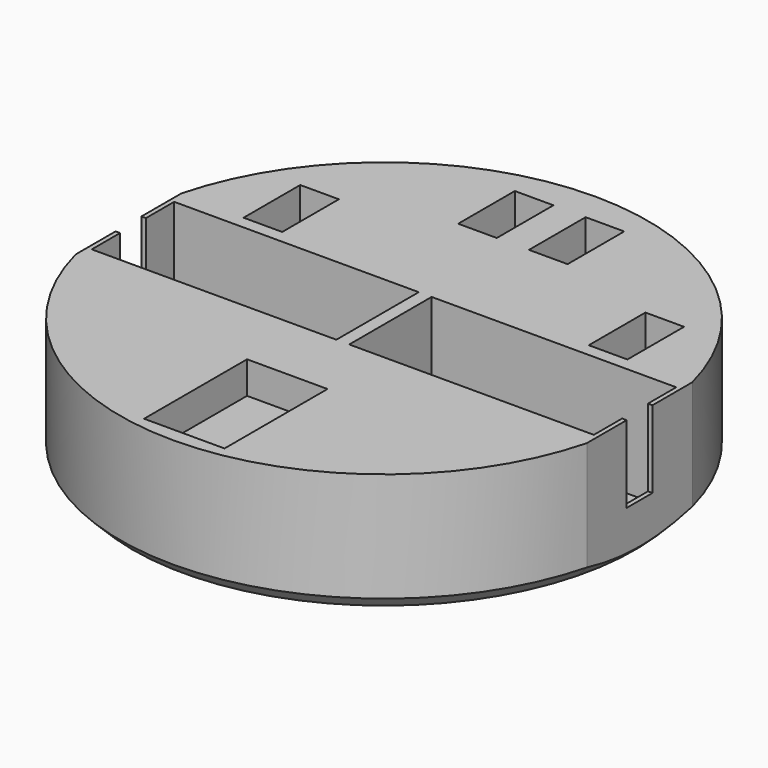
from build123d import *

# Parameters (mm, degrees)
F0_R        = 41
F1_DEPTH    = 19
F3_DEPTH    = 17
F4_W        = 6
F4_H        = 11
F4_W_2      = 11
F4_H_2      = 16
F4_W_3      = 10.7800960541
F4_H_3      = 45.1917052269
F5_DEPTH    = 19.001
F7_START    = -12
F6_W        = 0.7
F6_H        = 5
F7_DEPTH    = 5
F8_W        = 16
F8_H        = 16
F9_DEPTH    = 1.82
F10_C1_SIZE = 2
F10_C2_SIZE = 1.9999
F11_W       = 12.5
F11_H       = 20
F12_DEPTH   = 5
F13_W       = 6
F13_H       = 35
F14_DEPTH   = 28.5


# Not quite as in the source:
# - a fillet or chamfer is up to 0.001 mm smaller than in the source, because OpenCascade refuses the exact size


with BuildPart() as f1:
    # F0 (on Top) → F1 (new body)
    with BuildSketch(Plane.XY):
        Circle(F0_R)
    extrude(amount=F1_DEPTH)

    # F2 (on face) → F3 (cut)
    with BuildSketch(Plane.XY.offset(19)):
        Polygon((39, 2.5), (39, 8), (1, 8), (1, -8), (39, -8), (39, -2.5), align=None)
        Polygon((-39, 8), (-39, 2.5), (-39, -2.5), (-39, -8), (-1, -8), (-1, 8), align=None)
        with BuildLine():
            Line((43, 2.5), (40.9237095093, 2.5))
            ThreePointArc((40.9237095093, 2.5), (40.9809229391, 1.2505818885), (41, 0))
            ThreePointArc((41, 0), (40.9809229391, -1.2505818885), (40.9237095093, -2.5))
            Line((40.9237095093, -2.5), (43, -2.5))
            Line((43, -2.5), (43, 2.5))
        make_face()
        with BuildLine():
            ThreePointArc((-40.9237095093, -2.5), (-41, 0), (-40.9237095093, 2.5))
            Line((-40.9237095093, 2.5), (-43, 2.5))
            Line((-43, 2.5), (-43, -2.5))
            Line((-43, -2.5), (-40.9237095093, -2.5))
        make_face()
        with BuildLine():
            Line((40.9237095093, 2.5), (39, 2.5))
            Line((39, 2.5), (39, -2.5))
            Line((39, -2.5), (40.9237095093, -2.5))
            ThreePointArc((40.9237095093, -2.5), (40.9809229391, -1.2505818885), (41, 0))
            ThreePointArc((41, 0), (40.9809229391, 1.2505818885), (40.9237095093, 2.5))
        make_face()
        with BuildLine():
            Line((-39, 2.5), (-40.9237095093, 2.5))
            ThreePointArc((-40.9237095093, 2.5), (-41, 0), (-40.9237095093, -2.5))
            Line((-40.9237095093, -2.5), (-39, -2.5))
            Line((-39, -2.5), (-39, 2.5))
        make_face()
    extrude(amount=-F3_DEPTH, mode=Mode.SUBTRACT)

    # F4 (on face) → F5 (cut, through all)
    with BuildSketch(Plane.XY.offset(19)):
        with Locations((-26.8149985671, 15.5)):
            Rectangle(F4_W, F4_H)
        with Locations((26.8149985671, 15.5)):
            Rectangle(F4_W, F4_H)
        with Locations((-5.5, 30.5270385295)):
            Rectangle(F4_W, F4_H)
        with Locations((5.5, 30.5270385295)):
            Rectangle(F4_W, F4_H)
        with Locations((-6.5, 0)):
            Rectangle(F4_W_2, F4_H_2)
        with Locations((6.5, 0)):
            Rectangle(F4_W_2, F4_H_2)
        with Locations((-45.090048027, 0)):
            Rectangle(F4_W_3, F4_H_3)
        with Locations((45.090048027, 0)):
            Rectangle(F4_W_3, F4_H_3)
    extrude(amount=-F5_DEPTH, mode=Mode.SUBTRACT)

    # F6 (on face) → F7 (join)
    with BuildSketch(Plane.XY.offset(19).offset(F7_START)):
        with Locations((-39.35, 0)):
            Rectangle(F6_W, F6_H)
        with Locations((39.35, 0)):
            Rectangle(F6_W, F6_H)
    extrude(amount=-F7_DEPTH)

    # F8 (on face) → F9 (join)
    with BuildSketch(Plane.XY.offset(2)):
        with Locations((-20, 0)):
            Rectangle(F8_W, F8_H)
        with Locations((20, 0)):
            Rectangle(F8_W, F8_H)
    extrude(amount=F9_DEPTH)

    # F10: chamfer of 2 on 2 edges, made by hand

    # F10_c1
    f10_c1_edges = [f1.edges().sort_by_distance(p)[0] for p in [
        (0, -41, 0),
    ]]
    chamfer(f10_c1_edges, length=F10_C1_SIZE)

    # F10_c2 (size 2 in the source; OpenCascade refuses exactly that, so slightly less here)
    f10_c2_edges = [f1.edges().sort_by_distance(p)[0] for p in [
        (0, 41, 0),
    ]]
    chamfer(f10_c2_edges, length=F10_C2_SIZE)

    # F11 (on face) → F12 (cut)
    with BuildSketch(Plane.XY.offset(19)):
        with Locations((0, -28.7845470011)):
            Rectangle(F11_W, F11_H)
    extrude(amount=-F12_DEPTH, mode=Mode.SUBTRACT)

    # F13 (on Right) → F14 (cut, symmetric)
    with BuildSketch(Plane.YZ):
        with Locations((-14.7845470011, -0.5)):
            Rectangle(F13_W, F13_H)
    extrude(amount=F14_DEPTH, both=True, mode=Mode.SUBTRACT)


solid = f1.part
